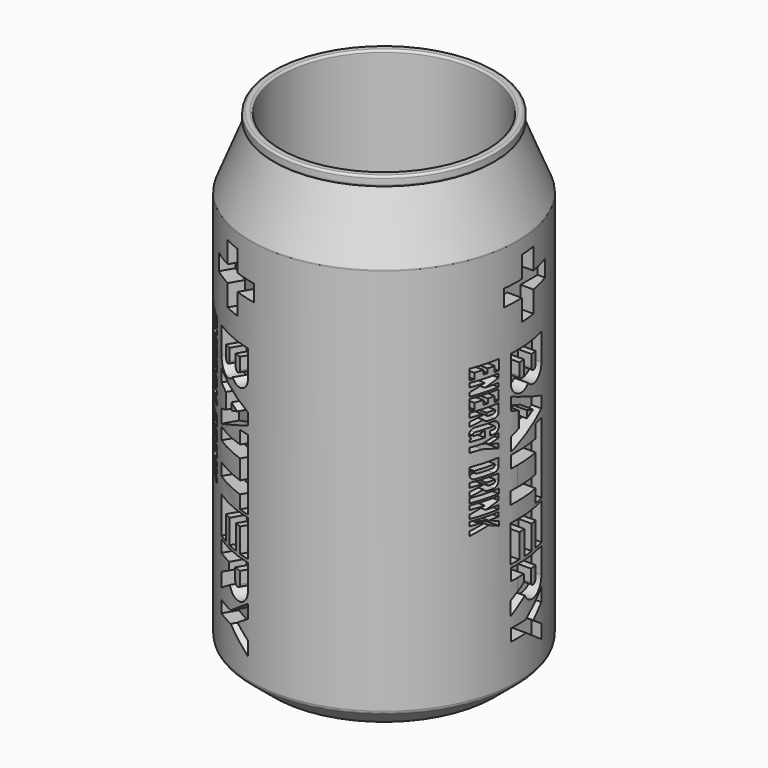
from build123d import *

# Parameters (mm, degrees)
F0_R             = 32.5
F1_DEPTH         = 115
F2_SIZE2         = 6
F2_SIZE          = 5
F3_R             = 1.0429426603
F5_R             = 25
F6_DEPTH         = 103.4
F7_R             = 27
F7_R_2           = 26.5
F7_R_3           = 25
F8_DEPTH         = 2.4
F9_R             = 0.49999
F11_W            = 6.676602
F11_H            = 1.102272
F12_DEPTH        = 12.3
F12_COPIES_COUNT = 3
F13_R            = 4.3455844123


# Not quite as in the source:
# - a fillet or chamfer that OpenCascade refuses, or shapes differently, is made with other operations: its cross-section is extruded or revolved along the edge and cut away or added
# - a fillet or chamfer is up to 0.001 mm smaller than in the source, because OpenCascade refuses the exact size
# - ends of sketch curves that miss each other by under 0.0002 mm in the source are joined
# - a pattern or mirror of a feature is missing from the dataset's text; its kind, count and spacing are read off the source's solid


with BuildPart() as f1:
    # F0 (on Top) → F1 (new body)
    with BuildSketch(Plane.XY):
        Circle(F0_R)
    extrude(amount=F1_DEPTH)

    # F2
    f2_edges = [f1.edges().sort_by_distance(p)[0] for p in [
        (-32.5, 0, 0),
    ]]
    chamfer(f2_edges, length=F2_SIZE, length2=F2_SIZE2)

    # F3
    f3_edges = [f1.edges().sort_by_distance(p)[0] for p in [
        (-32.5, 0, 5),
        (-26.5, 0, 0),
    ]]
    fillet(f3_edges, radius=F3_R)

    # F4: chamfer of 6 x 15 on 1 edges, made by hand

    # F4_s1 → F4_t2 (revolve, cut)
    with BuildSketch(Plane.XZ):
        Polygon((32.5, 100), (26.5, 115), (32.5, 115), align=None)
    revolve(axis=Axis((0, 0, 115), (0, 0, 1)), mode=Mode.SUBTRACT)

    # F5 (on face) → F6 (cut)
    with BuildSketch(Plane.XY.offset(115)):
        Circle(F5_R)
    extrude(amount=-F6_DEPTH, mode=Mode.SUBTRACT)

    # F7 (on face) → F8 (join)
    with BuildSketch(Plane.XY.offset(115)):
        Circle(F7_R)
        Circle(F7_R_2, mode=Mode.SUBTRACT)
        Circle(F7_R_2)
        Circle(F7_R_3, mode=Mode.SUBTRACT)
    extrude(amount=F8_DEPTH)

    # F9 (radius 0.5 in the source; OpenCascade refuses exactly that, so slightly less here)
    f9_edges = [f1.edges().sort_by_distance(p)[0] for p in [
        (27, 0, 116.2),
        (-27, 0, 115),
        (-27, 0, 117.4),
        (-25, 0, 117.4),
        (-32.5, 0, 100),
    ]]
    fillet(f9_edges, radius=F9_R)

    # F11 (on offset) → F12 (cut)
    with BuildSketch(Plane.YZ.offset(41.2)):
        Polygon((-11.779934193, 42.8567660874), (-9.718265193, 42.8567660874), (-9.001789193, 42.5073220874), (-11.790930193, 41.8297040874), (-11.790930193, 40.7671540874), (-7.607217193, 41.8539930874), (-5.137932193, 40.8674810874), (-5.137932193, 41.9044210874), (-7.607217193, 42.8567660874), (-5.211895193, 42.8567660874), (-5.211895193, 43.8504450874), (-11.779934193, 43.8504450874), align=None)
        Polygon((-6.166673193, 67.7603460874), (-5.175054193, 67.7603460874), (-5.175054193, 69.0884540874), (-5.175054193, 70.1917200874), (-11.815032193, 70.1917200874), (-11.815032193, 69.1268360874), (-11.815032193, 69.0884540874), (-11.815030193, 67.6515530874), (-10.791918193, 67.6515530874), (-10.791918193, 69.0884540874), (-8.845362193, 69.0884540874), (-8.845362193, 68.0432200874), (-7.806563193, 68.0432200874), (-7.806563193, 69.0884540874), (-6.166673193, 69.0884540874), align=None)
        Polygon((-7.833460193, 74.5382150874), (-7.833460193, 75.5514660874), (-6.193570193, 75.5514660874), (-6.193570193, 74.1849760874), (-5.156716193, 74.1849760874), (-5.156716193, 75.5514660874), (-5.156716193, 76.6675240874), (-11.822736193, 76.6675240874), (-11.822736193, 75.5514660874), (-11.822736193, 74.1401510874), (-10.818814193, 74.1401510874), (-10.818814193, 75.5514660874), (-8.846671193, 75.5514660874), (-8.846671193, 74.5382150874), align=None)
        Polygon((-8.493857193, 72.6564630874), (-11.795840193, 71.6070230874), (-11.795840193, 70.6661470874), (-5.191873193, 70.6661470874), (-5.191873193, 71.6070230874), (-8.493857193, 71.6070230874), (-5.191873193, 72.6564630874), (-5.191873193, 73.5973390874), (-11.805299193, 73.5973390874), (-11.805299193, 72.6564630874), align=None)
        Polygon((2.765040807, 14.7856650874), (8.833066807, 10.6109970874), (8.833066807, 13.9758800874), (5.417141807, 16.3044290874), (8.820272807, 18.5562100874), (8.820272807, 21.8059470874), (2.765040807, 17.6904900874), (-1.925533193, 17.6904900874), (-1.925533193, 14.7856650874), align=None)
        Polygon((4.791350807, 31.4185650874), (4.791350807, 37.3102130874), (6.329077807, 37.3102130874), (6.329077807, 31.4209210874), (8.853059807, 31.4209210874), (8.853059807, 37.3102130874), (8.853059807, 40.2813930874), (-1.978389193, 40.2813930874), (-1.978389193, 37.3102130874), (-1.978389193, 31.4282520874), (0.594602807, 31.4282520874), (0.594602807, 37.3102130874), (2.252159807, 37.3102130874), (2.252159807, 31.4185650874), align=None)
        with BuildLine():
            Line((-1.915084193, 27.7547050874), (2.042059807, 27.7547050874))
            Line((2.042059807, 27.7547050874), (2.042059807, 25.8986850874))
            Line((2.042059807, 25.8986850874), (-1.975169193, 23.6596940874))
            Line((-1.975169193, 23.6596940874), (-1.975169193, 20.2948140874))
            Line((-1.975169193, 20.2948140874), (2.361902807, 22.9432160874))
            ThreePointArc((2.361902807, 22.9432160874), (6.2150620717, 21.1316307787), (8.859399807, 24.4687190874))
            Line((8.859399807, 24.4687190874), (8.859399807, 27.7547050874))
            Line((8.859399807, 27.7547050874), (8.859399807, 30.6474930874))
            Line((8.859399807, 30.6474930874), (-1.915084193, 30.6474930874))
            Line((-1.915084193, 30.6474930874), (-1.915084193, 27.7547050874))
        make_face()
        with BuildLine():
            ThreePointArc((6.275067807, 24.8397510874), (5.424284807, 23.9889680874), (4.573501807, 24.8397510874))
            Line((4.573501807, 24.8397510874), (4.573501807, 27.7547050874))
            Line((4.573501807, 27.7547050874), (6.275066807, 27.7547050874))
            Line((6.275066807, 27.7547050874), (6.275067807, 24.8397510874))
        make_face(mode=Mode.SUBTRACT)
        Polygon((6.306709807, 58.0855600874), (6.306709807, 54.8605080874), (-1.937907193, 54.8605080874), (-1.937907193, 51.9018280874), (6.306709807, 51.9018280874), (6.306709807, 47.1852760874), (-1.978389193, 47.1852760874), (-1.978389193, 44.1920370874), (6.306709807, 44.1920370874), (6.306709807, 40.9681610874), (8.850607807, 40.9681610874), (8.850607807, 58.0855600874), align=None)
        Polygon((8.860835807, 60.0917500874), (8.860835807, 62.9063700874), (-1.899469193, 67.3835260874), (-1.899469193, 64.3257980874), (0.479767807, 63.4392390874), (0.479767807, 59.6626170874), (-1.899469193, 58.7036850874), (-1.899469193, 55.4830430874), align=None)
        Polygon((3.045376807, 62.4360570874), (5.343194807, 61.5494970874), (3.045376807, 60.6629370874), align=None, mode=Mode.SUBTRACT)
        with BuildLine():
            Line((-5.186217193, 67.2112010874), (-11.799490193, 67.2112010874))
            Line((-11.799490193, 67.2112010874), (-11.799490193, 66.1346640874))
            Line((-11.799490193, 66.1346640874), (-9.058283193, 66.1346640874))
            Line((-9.058283193, 66.1346640874), (-9.058283193, 65.8723150874))
            Line((-9.058283193, 65.8723150874), (-11.808537193, 65.2571510874))
            Line((-11.808537193, 65.2571510874), (-11.808537193, 64.1806150874))
            Line((-11.808537193, 64.1806150874), (-8.841158193, 64.8591040874))
            ThreePointArc((-8.841158193, 64.8591040874), (-8.4348090344, 64.4422366447), (-7.873142193, 64.2891720874))
            Line((-7.873142193, 64.2891720874), (-6.181374193, 64.2891720874))
            ThreePointArc((-6.181374193, 64.2891720874), (-5.4708630377, 64.6611580139), (-5.186217193, 65.4109420874))
            Line((-5.186217193, 65.4109420874), (-5.186217193, 66.1346640874))
            Line((-5.186217193, 66.1346640874), (-5.186217193, 67.2112010874))
        make_face()
        with BuildLine():
            Line((-8.099313193, 66.1346640874), (-6.108999193, 66.1346640874))
            Line((-6.108999193, 66.1346640874), (-6.108999193, 65.7456640874))
            ThreePointArc((-6.108999193, 65.7456640874), (-6.2509413423, 65.4434600953), (-6.561344193, 65.3204770874))
            Line((-6.561344193, 65.3204770874), (-7.583642193, 65.3204770874))
            ThreePointArc((-7.583642193, 65.3204770874), (-7.9417288288, 65.4114852582), (-8.099314193, 65.7456640874))
            Line((-8.099314193, 65.7456640874), (-8.099313193, 66.1346640874))
        make_face(mode=Mode.SUBTRACT)
        with BuildLine():
            ThreePointArc((-6.501624193, 60.9410430874), (-5.0984757837, 62.4174720544), (-6.6443631261, 63.7437074323))
            Line((-6.6443631261, 63.7437074323), (-10.671064193, 63.7623700874))
            ThreePointArc((-10.671064193, 63.7623700874), (-11.839685668, 62.9042184154), (-11.3580081595, 61.5367071369))
            Line((-11.3580081595, 61.5367071369), (-11.787972193, 61.3369530874))
            Line((-11.787972193, 61.3369530874), (-11.787972193, 60.9147610874))
            Line((-11.787972193, 60.9147610874), (-10.751640193, 60.9147610874))
            Line((-10.751640193, 60.9147610874), (-9.331481193, 60.9147610874))
            Line((-9.331481193, 60.9147610874), (-8.487960193, 60.9147610874))
            Line((-8.487960193, 60.9147610874), (-8.487960193, 62.3241140874))
            Line((-8.487960193, 62.3241140874), (-9.332379193, 62.3241140874))
            Line((-9.332379193, 62.3241140874), (-9.332379193, 61.9786840874))
            Line((-9.332379193, 61.9786840874), (-10.752539193, 61.9786840874))
            ThreePointArc((-10.752539193, 61.9786840874), (-11.130274193, 62.3564190874), (-10.752539193, 62.7341540874))
            Line((-10.752539193, 62.7341540874), (-6.372830193, 62.7138550874))
            ThreePointArc((-6.372830193, 62.7138550874), (-6.002838193, 62.3438630874), (-6.372830193, 61.9738710874))
            Line((-6.372830193, 61.9738710874), (-7.259714193, 61.9738710874))
            Line((-7.259714193, 61.9738710874), (-7.259714193, 60.9410430874))
            Line((-7.259714193, 60.9410430874), (-6.501624193, 60.9410430874))
        make_face()
        Polygon((-9.138212193, 59.7560440874), (-11.795591193, 59.7560440874), (-11.795591193, 58.6156760874), (-9.138212193, 58.6156760874), (-5.179040193, 57.5183400874), (-5.179040193, 58.5618850874), (-7.492143193, 59.2073770874), (-5.211316193, 59.7560440874), (-5.211316193, 60.7995890874), align=None)
        with BuildLine():
            Line((-5.178054193, 54.4842620874), (-5.178054193, 55.5202190874))
            Line((-5.178054193, 55.5202190874), (-11.795840193, 55.5202190874))
            Line((-11.795840193, 55.5202190874), (-11.795840193, 54.4842620874))
            Line((-11.795840193, 54.4842620874), (-11.795840193, 53.8311200874))
            ThreePointArc((-11.795840193, 53.8311200874), (-11.5133454009, 53.0666897025), (-10.8016362386, 52.669666795))
            Line((-10.8016362386, 52.669666795), (-6.425683193, 52.6696670874))
            ThreePointArc((-6.425683193, 52.6696670874), (-5.5502102137, 52.9681039068), (-5.178055193, 53.8148730874))
            Line((-5.178055193, 53.8148730874), (-5.178054193, 54.4842620874))
        make_face()
        with BuildLine():
            Line((-10.838029193, 54.4842620874), (-6.104300193, 54.4842620874))
            ThreePointArc((-6.104300193, 54.4842620874), (-6.2978244686, 53.9592441596), (-6.811913193, 53.7383180874))
            Line((-6.811913193, 53.7383180874), (-10.153355193, 53.7383180874))
            ThreePointArc((-10.153355193, 53.7383180874), (-10.6596185825, 53.9608281153), (-10.838029193, 54.4842620874))
        make_face(mode=Mode.SUBTRACT)
        with BuildLine():
            Line((-5.223699193, 51.1337410874), (-5.223699193, 52.1668990874))
            Line((-5.223699193, 52.1668990874), (-11.811788193, 52.1668990874))
            Line((-11.811788193, 52.1668990874), (-11.811788193, 51.1337410874))
            Line((-11.811788193, 51.1337410874), (-9.012230193, 51.1337410874))
            Line((-9.012230193, 51.1337410874), (-9.012230193, 50.8588580874))
            Line((-9.012230193, 50.8588580874), (-11.796573193, 50.2659710874))
            Line((-11.796573193, 50.2659710874), (-11.796573193, 49.1546120874))
            Line((-11.796573193, 49.1546120874), (-8.814436193, 49.8692100874))
            ThreePointArc((-8.814436193, 49.8692100874), (-8.3661282094, 49.4608534309), (-7.778012193, 49.3130200874))
            Line((-7.778012193, 49.3130200874), (-6.235406193, 49.3130200874))
            ThreePointArc((-6.235406193, 49.3130200874), (-5.5054492469, 49.8061108441), (-5.223699193, 50.6407320874))
            Line((-5.223699193, 50.6407320874), (-5.223699193, 51.1337410874))
        make_face()
        with BuildLine():
            Line((-8.105873193, 51.1337410874), (-6.061735193, 51.1337410874))
            Line((-6.061735193, 51.1337410874), (-6.061735193, 50.8239890874))
            ThreePointArc((-6.061735193, 50.8239890874), (-6.2354063652, 50.492735869), (-6.585101193, 50.3600560874))
            Line((-6.585101193, 50.3600560874), (-7.594611193, 50.3600560874))
            ThreePointArc((-7.594611193, 50.3600560874), (-7.9328730888, 50.486230367), (-8.105872799, 50.803109144))
            Line((-8.105872799, 50.803109144), (-8.105873193, 51.1337410874))
        make_face(mode=Mode.SUBTRACT)
        with Locations((-8.472145193, 48.3195640874)):
            Rectangle(F11_W, F11_H)
        Polygon((-5.188125193, 46.3562830874), (-5.188125193, 47.3137360874), (-11.810446193, 47.3137360874), (-11.810446193, 46.3562830874), (-8.499286193, 46.3562830874), (-11.792351193, 45.3584570874), (-11.792351193, 44.4191020874), (-5.188125193, 44.4191020874), (-5.188125193, 45.3584570874), (-8.282160193, 45.3584570874), align=None)
        Polygon((10.667086807, 87.2374990874), (10.667086807, 91.2835440874), (5.458859807, 91.2835440874), (5.458859807, 96.4729370874), (1.397946807, 96.4729370874), (1.397946807, 91.2835440874), (-3.784830193, 91.2835440874), (-3.784830193, 87.2374990874), (1.397946807, 87.2374990874), (1.397946807, 82.0355300874), (5.458859807, 82.0355300874), (5.458859807, 87.2374990874), align=None)
        with BuildLine():
            Line((8.888406807, 70.1128940874), (8.888406807, 76.6101210874))
            Line((8.888406807, 76.6101210874), (-1.901924193, 76.6101210874))
            Line((-1.901924193, 76.6101210874), (-1.901924193, 70.1128940874))
            ThreePointArc((-1.901924193, 70.1128940874), (0.1058976523, 67.2025530234), (3.5395067213, 68.0462131635))
            ThreePointArc((3.5395067213, 68.0462131635), (6.9224898673, 67.2457568559), (8.888406807, 70.1128940874))
        make_face()
        with BuildLine():
            Line((0.630953807, 73.7028640874), (2.156482807, 73.7028640874))
            Line((2.156482807, 73.7028640874), (2.156482807, 70.7743360874))
            ThreePointArc((2.156482807, 70.7743360874), (1.393717807, 70.0115720874), (0.630953807, 70.7743360874))
            Line((0.630953807, 70.7743360874), (0.630953807, 73.7028640874))
        make_face(mode=Mode.SUBTRACT)
        with BuildLine():
            ThreePointArc((6.282730807, 70.7743360874), (5.519966807, 70.0115720874), (4.757202807, 70.7743360874))
            Line((4.757202807, 70.7743360874), (4.757202807, 73.7028640874))
            Line((4.757202807, 73.7028640874), (6.282730807, 73.7028640874))
            Line((6.282730807, 73.7028640874), (6.282730807, 70.7743360874))
        make_face(mode=Mode.SUBTRACT)
    f12 = extrude(amount=-F12_DEPTH, mode=Mode.SUBTRACT)

    # F12_copies: F12 ×3 about axis
    f12_copies_axis = Axis((0, 0, 0), (0, 0, 1))
    for i in range(1, F12_COPIES_COUNT):
        add(f12.rotate(f12_copies_axis, i * 360 / F12_COPIES_COUNT), mode=Mode.SUBTRACT)

    # F13
    f13_edges = [f1.edges().sort_by_distance(p)[0] for p in [
        (-25, 0, 11.6),
    ]]
    fillet(f13_edges, radius=F13_R)


solid = f1.part
